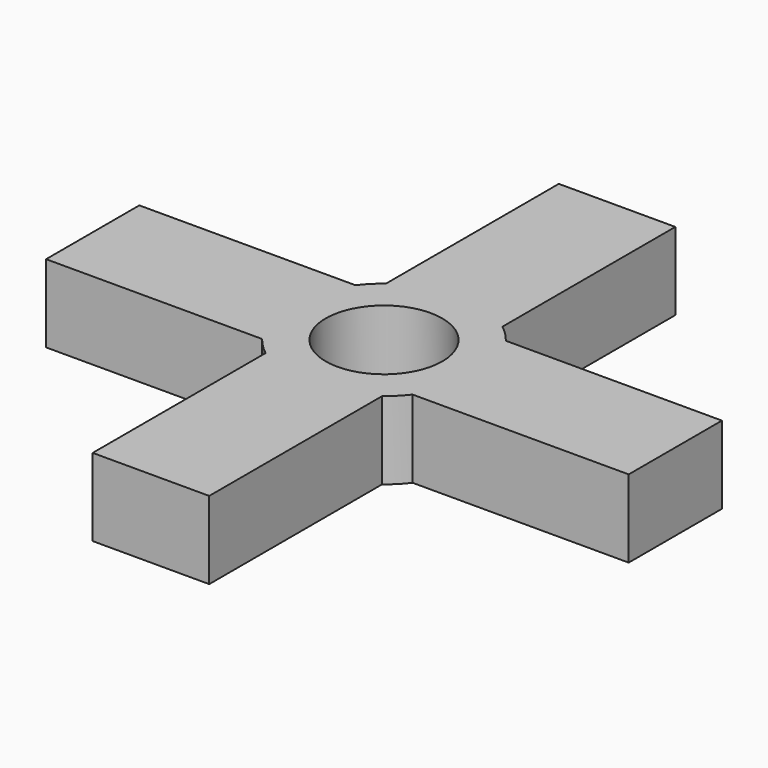
from build123d import *

# Parameters (mm, degrees)
F0_W     = 3
F0_H     = 3
F1_DEPTH = 2
F2_R     = 1.5
F3_DEPTH = 2.001


with BuildPart() as f1:
    # F0 (on Top) → F1 (new body)
    with BuildSketch(Plane.XY):
        with BuildLine():
            ThreePointArc((-1.9371370628, -1.5), (-2.45, 0), (-1.9371370628, 1.5))
            Line((-1.9371370628, 1.5), (-7.5, 1.5))
            Line((-7.5, 1.5), (-7.5, -1.5))
            Line((-7.5, -1.5), (-1.9371370628, -1.5))
        make_face()
        Rectangle(F0_W, F0_H)
        with BuildLine():
            Line((-1.5, -1.5), (-1.5, 1.5))
            Line((-1.5, 1.5), (-1.9371370628, 1.5))
            ThreePointArc((-1.9371370628, 1.5), (-2.45, 0), (-1.9371370628, -1.5))
            Line((-1.9371370628, -1.5), (-1.5, -1.5))
        make_face()
        with BuildLine():
            ThreePointArc((1.9371370628, 1.5), (2.3182413381, 0.7926267079), (2.45, 0))
            ThreePointArc((2.45, 0), (2.3182413381, -0.7926267079), (1.9371370628, -1.5))
            Line((1.9371370628, -1.5), (7.5, -1.5))
            Line((7.5, -1.5), (7.5, 1.5))
            Line((7.5, 1.5), (1.9371370628, 1.5))
        make_face()
        with BuildLine():
            Line((1.5, -7.5), (1.5, -1.9371370628))
            ThreePointArc((1.5, -1.9371370628), (0, -2.45), (-1.5, -1.9371370628))
            Line((-1.5, -1.9371370628), (-1.5, -7.5))
            Line((-1.5, -7.5), (1.5, -7.5))
        make_face()
        with BuildLine():
            Line((1.5, 1.5), (1.5, 1.9371370628))
            ThreePointArc((1.5, 1.9371370628), (0, 2.45), (-1.5, 1.9371370628))
            Line((-1.5, 1.9371370628), (-1.5, 1.5))
            Line((-1.5, 1.5), (1.5, 1.5))
        make_face()
        with BuildLine():
            ThreePointArc((1.9371370628, -1.5), (2.3182413381, -0.7926267079), (2.45, 0))
            ThreePointArc((2.45, 0), (2.3182413381, 0.7926267079), (1.9371370628, 1.5))
            Line((1.9371370628, 1.5), (1.5, 1.5))
            Line((1.5, 1.5), (1.5, -1.5))
            Line((1.5, -1.5), (1.9371370628, -1.5))
        make_face()
        with BuildLine():
            ThreePointArc((-1.5, 1.9371370628), (0, 2.45), (1.5, 1.9371370628))
            Line((1.5, 1.9371370628), (1.5, 7.5))
            Line((1.5, 7.5), (-1.5, 7.5))
            Line((-1.5, 7.5), (-1.5, 1.9371370628))
        make_face()
        with BuildLine():
            ThreePointArc((-1.5, -1.9371370628), (0, -2.45), (1.5, -1.9371370628))
            Line((1.5, -1.9371370628), (1.5, -1.5))
            Line((1.5, -1.5), (-1.5, -1.5))
            Line((-1.5, -1.5), (-1.5, -1.9371370628))
        make_face()
        with BuildLine():
            ThreePointArc((-1.9371370628, -1.5), (-1.7324116139, -1.7324116139), (-1.5, -1.9371370628))
            Line((-1.5, -1.9371370628), (-1.5, -1.5))
            Line((-1.5, -1.5), (-1.9371370628, -1.5))
        make_face()
        with BuildLine():
            Line((1.5, 1.5), (1.9371370628, 1.5))
            ThreePointArc((1.9371370628, 1.5), (1.7324116139, 1.7324116139), (1.5, 1.9371370628))
            Line((1.5, 1.9371370628), (1.5, 1.5))
        make_face()
        with BuildLine():
            ThreePointArc((1.5, -1.9371370628), (1.7324116139, -1.7324116139), (1.9371370628, -1.5))
            Line((1.9371370628, -1.5), (1.5, -1.5))
            Line((1.5, -1.5), (1.5, -1.9371370628))
        make_face()
        with BuildLine():
            Line((-1.5, 1.5), (-1.5, 1.9371370628))
            ThreePointArc((-1.5, 1.9371370628), (-1.7324116139, 1.7324116139), (-1.9371370628, 1.5))
            Line((-1.9371370628, 1.5), (-1.5, 1.5))
        make_face()
    extrude(amount=F1_DEPTH)

    # F2 (on face) → F3 (cut, through all)
    with BuildSketch(Plane.XY.offset(2)):
        Circle(F2_R)
    extrude(amount=-F3_DEPTH, mode=Mode.SUBTRACT)


solid = f1.part
